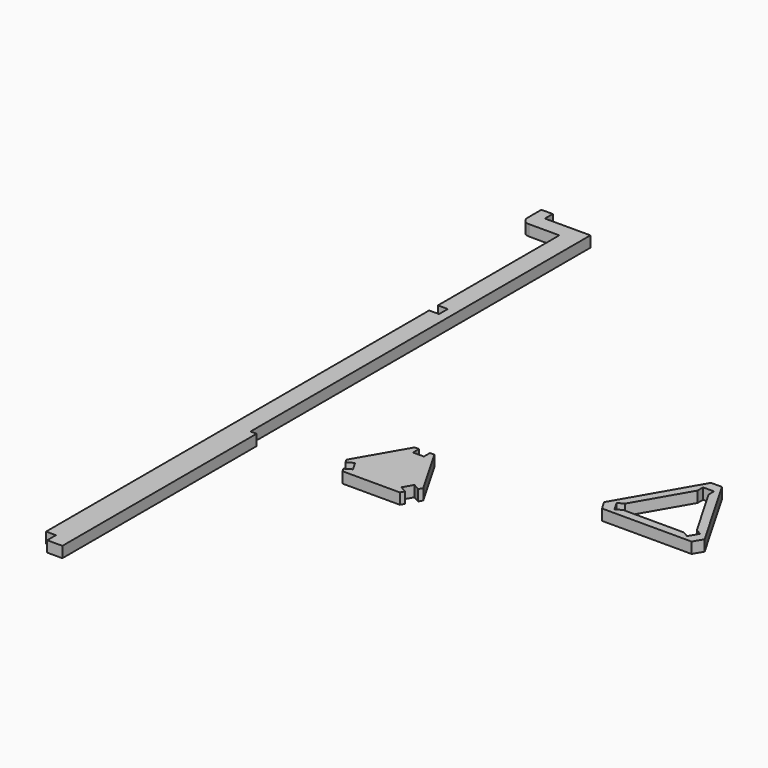
from build123d import *

# Parameters (mm, degrees)
F1_W     = 44.45
F1_H     = 25.4
F2_DEPTH = 18.288


# Not quite as in the source:
# - a variable given as a bare number and used for a length is read in inches; the dataset says mm whatever the document's units were


with BuildPart() as f2:
    # F1 (on Top) → F2 (new body)
    with BuildSketch(Plane.XY):
        Polygon((0, 413.512), (0, 0), (31.75, 0), (31.75, 685.8), (0, 685.8), (0, 431.8), (16.51, 431.8), (16.51, 413.512), align=None)
        Polygon((31.75, 0), (0, 0), (0, -388.112), (16.51, -388.112), (16.51, -406.4), (41.91, -406.4), (41.91, 0), align=None)
        with BuildLine():
            Line((-50.8, 685.8), (-44.45, 685.8))
            Line((-44.45, 685.8), (-44.45, 711.2))
            Line((-44.45, 711.2), (-44.45, 727.71))
            Line((-44.45, 727.71), (-63.5, 727.71))
            Line((-63.5, 727.71), (-63.5, 698.5))
            ThreePointArc((-63.5, 698.5), (-59.7802561211, 689.5197438789), (-50.8, 685.8))
        make_face()
        Polygon((0, 685.8), (31.75, 685.8), (31.75, 711.2), (12.7, 711.2), (0, 711.2), align=None)
        with Locations((-22.225, 698.5)):
            Rectangle(F1_W, F1_H)
    extrude(amount=F2_DEPTH)


with BuildPart() as f2b:
    # F1 (on Top) → F2, piece 2 (new body)
    with BuildSketch(Plane.XY):
        Polygon((252.984, 98.928417404), (252.984, 86.228417404), (293.624, 15.8378725844), (304.6225226281, 9.4878725844), (308.2886968374, 15.8378725844), (260.3163484187, 98.928417404), align=None)
        Polygon((234.696, 86.228417404), (194.056, 15.8378725844), (203.2, 0), (284.48, 0), (293.624, 15.8378725844), (252.984, 86.228417404), align=None)
        Polygon((284.48, 0), (203.2, 0), (192.2014773719, -6.35), (195.8676515813, -12.7), (291.8123484187, -12.7), (295.4785226281, -6.35), align=None)
        Polygon((183.0574773719, 9.4878725844), (194.056, 15.8378725844), (234.696, 86.228417404), (234.696, 98.928417404), (227.3636515813, 98.928417404), (179.3913031626, 15.8378725844), align=None)
    extrude(amount=F2_DEPTH)


with BuildPart() as f2c:
    # F1 (on Top) → F2, piece 3 (new body)
    with BuildSketch(Plane.XY):
        Polygon((592.5288027261, 262.5760536089), (517.5320529443, 132.6778725844), (526.6760529443, 116.84), (676.6695525078, 116.84), (685.8135525078, 132.6778725844), (610.8168027261, 262.5760536089), align=None)
        Polygon((531.8301323608, 140.9328725844), (541.7288027261, 146.6478725844), (592.5288027261, 234.6360536089), (592.5288027261, 246.0660536089), (610.8168027261, 246.0660536089), (610.8168027261, 234.6360536089), (661.6168027261, 146.6478725844), (671.5154730913, 140.9328725844), (662.3714730913, 125.095), (652.4728027261, 130.81), (550.8728027261, 130.81), (540.9741323608, 125.095), align=None, mode=Mode.SUBTRACT)
    extrude(amount=F2_DEPTH)


solid = Compound([f2.part, f2b.part, f2c.part])
